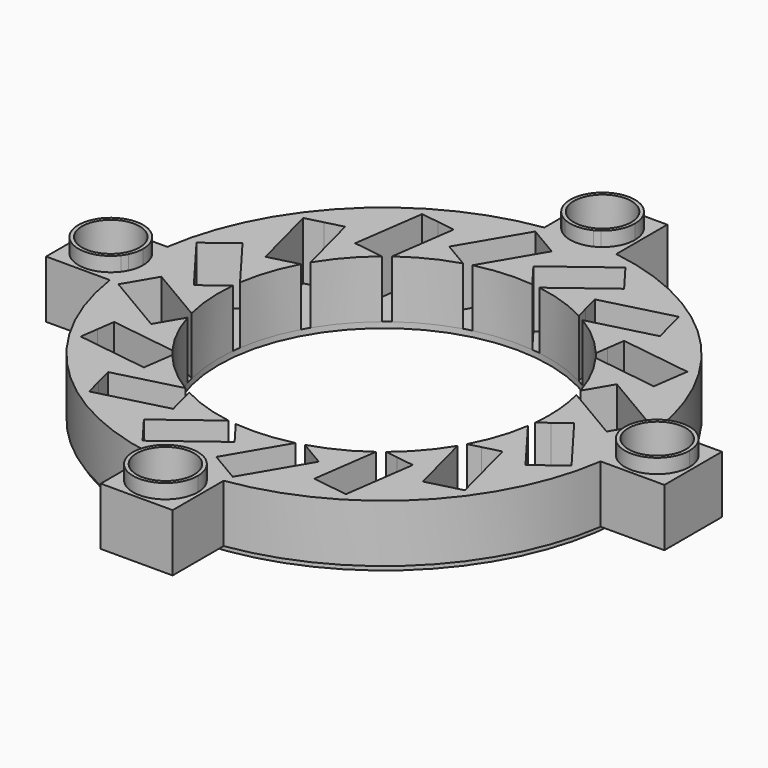
from build123d import *

# Parameters (mm, degrees)
F1_R     = 23
F2_DEPTH = 8
F1_R_2   = 4
F3_DEPTH = 10
F4_DEPTH = 0.8
F5_DEPTH = 25


# Not quite as in the source:
# - a feature names something its author has since deleted; it is built from what else it names


with BuildPart() as f2:
    # F1 (on Top) → F2 (new body)
    with BuildSketch(Plane.XY):
        with BuildLine():
            ThreePointArc((-33.9440789474, -1.9492317499), (-34.1514000153, -2.3320116118), (-34.3947368421, -2.6929681696))
            ThreePointArc((-34.3947368421, -2.6929681696), (-34.2846582705, -3.8486630504), (-34.1357583774, -5))
            ThreePointArc((-34.1357583774, -5), (-24.3951839509, -24.3951839509), (-5, -34.1357583774))
            ThreePointArc((-5, -34.1357583774), (-3.8486630504, -34.2846582705), (-2.6929681696, -34.3947368421))
            ThreePointArc((-2.6929681696, -34.3947368421), (-2.3320116118, -34.1514000153), (-1.9492317499, -33.9440789474))
            ThreePointArc((-1.9492317499, -33.9440789474), (-24.0416305603, -24.0416305603), (-33.9440789474, -1.9492317499))
        make_face()
        with BuildLine():
            ThreePointArc((-34.1357583774, -5), (-34.2846582705, -3.8486630504), (-34.3947368421, -2.6929681696))
            ThreePointArc((-34.3947368421, -2.6929681696), (-42.5, 0), (-34.3947368421, 2.6929681696))
            ThreePointArc((-34.3947368421, 2.6929681696), (-34.2846582705, 3.8486630504), (-34.1357583774, 5))
            Line((-34.1357583774, 5), (-43, 5))
            Line((-43, 5), (-43, 0))
            Line((-43, 0), (-43, -5))
            Line((-43, -5), (-34.1357583774, -5))
        make_face()
        with BuildLine():
            ThreePointArc((-34.1357583774, 5), (-34.2846582705, 3.8486630504), (-34.3947368421, 2.6929681696))
            ThreePointArc((-34.3947368421, 2.6929681696), (-34.1514000153, 2.3320116118), (-33.9440789474, 1.9492317499))
            ThreePointArc((-33.9440789474, 1.9492317499), (-24.0416305603, 24.0416305603), (-1.9492317499, 33.9440789474))
            ThreePointArc((-1.9492317499, 33.9440789474), (-2.3320116118, 34.1514000153), (-2.6929681696, 34.3947368421))
            ThreePointArc((-2.6929681696, 34.3947368421), (-3.8486630504, 34.2846582705), (-5, 34.1357583774))
            ThreePointArc((-5, 34.1357583774), (-24.3951839509, 24.3951839509), (-34.1357583774, 5))
        make_face()
        with BuildLine():
            ThreePointArc((-2.6929681696, -34.3947368421), (-3.8486630504, -34.2846582705), (-5, -34.1357583774))
            Line((-5, -34.1357583774), (-5, -43))
            Line((-5, -43), (0, -43))
            Line((0, -43), (5, -43))
            Line((5, -43), (5, -34.1357583774))
            ThreePointArc((5, -34.1357583774), (3.8486630504, -34.2846582705), (2.6929681696, -34.3947368421))
            ThreePointArc((2.6929681696, -34.3947368421), (4.022956423, -35.9836117392), (4.5, -38))
            ThreePointArc((4.5, -38), (-2.0163882608, -42.022956423), (-2.6929681696, -34.3947368421))
        make_face()
        with BuildLine():
            Line((-5, 43), (-5, 34.1357583774))
            ThreePointArc((-5, 34.1357583774), (-3.8486630504, 34.2846582705), (-2.6929681696, 34.3947368421))
            ThreePointArc((-2.6929681696, 34.3947368421), (-4.2704615799, 39.4188579544), (0, 42.5))
            Line((0, 42.5), (0, 43))
            Line((0, 43), (-5, 43))
        make_face()
        with BuildLine():
            ThreePointArc((33.9440789474, -1.9492317499), (24.0416305603, -24.0416305603), (1.9492317499, -33.9440789474))
            ThreePointArc((1.9492317499, -33.9440789474), (2.3320116118, -34.1514000153), (2.6929681696, -34.3947368421))
            ThreePointArc((2.6929681696, -34.3947368421), (3.8486630504, -34.2846582705), (5, -34.1357583774))
            ThreePointArc((5, -34.1357583774), (24.3951839509, -24.3951839509), (34.1357583774, -5))
            ThreePointArc((34.1357583774, -5), (34.2846582705, -3.8486630504), (34.3947368421, -2.6929681696))
            ThreePointArc((34.3947368421, -2.6929681696), (34.1514000153, -2.3320116118), (33.9440789474, -1.9492317499))
        make_face()
        with BuildLine():
            ThreePointArc((2.6929681696, 34.3947368421), (2.3320116118, 34.1514000153), (1.9492317499, 33.9440789474))
            ThreePointArc((1.9492317499, 33.9440789474), (24.0416305603, 24.0416305603), (33.9440789474, 1.9492317499))
            ThreePointArc((33.9440789474, 1.9492317499), (34.1514000153, 2.3320116118), (34.3947368421, 2.6929681696))
            ThreePointArc((34.3947368421, 2.6929681696), (34.2846582705, 3.8486630504), (34.1357583774, 5))
            ThreePointArc((34.1357583774, 5), (24.3951839509, 24.3951839509), (5, 34.1357583774))
            ThreePointArc((5, 34.1357583774), (3.8486630504, 34.2846582705), (2.6929681696, 34.3947368421))
        make_face()
        with BuildLine():
            Line((0, 43), (0, 42.5))
            ThreePointArc((0, 42.5), (3.1819805153, 41.1819805153), (4.5, 38))
            ThreePointArc((4.5, 38), (4.022956423, 35.9836117392), (2.6929681696, 34.3947368421))
            ThreePointArc((2.6929681696, 34.3947368421), (3.8486630504, 34.2846582705), (5, 34.1357583774))
            Line((5, 34.1357583774), (5, 43))
            Line((5, 43), (0, 43))
        make_face()
        with BuildLine():
            ThreePointArc((42.5, 0), (39.4188579544, -4.2704615799), (34.3947368421, -2.6929681696))
            ThreePointArc((34.3947368421, -2.6929681696), (34.2846582705, -3.8486630504), (34.1357583774, -5))
            Line((34.1357583774, -5), (43, -5))
            Line((43, -5), (43, 0))
            Line((43, 0), (43, 5))
            Line((43, 5), (34.1357583774, 5))
            ThreePointArc((34.1357583774, 5), (34.2846582705, 3.8486630504), (34.3947368421, 2.6929681696))
            ThreePointArc((34.3947368421, 2.6929681696), (39.4188579544, 4.2704615799), (42.5, 0))
        make_face()
        with BuildLine():
            ThreePointArc((-33.5, 0), (-33.6124240897, -0.9995887312), (-33.9440789474, -1.9492317499))
            ThreePointArc((-33.9440789474, -1.9492317499), (-24.0416305603, -24.0416305603), (-1.9492317499, -33.9440789474))
            ThreePointArc((-1.9492317499, -33.9440789474), (0, -33.5), (1.9492317499, -33.9440789474))
            ThreePointArc((1.9492317499, -33.9440789474), (24.0416305603, -24.0416305603), (33.9440789474, -1.9492317499))
            ThreePointArc((33.9440789474, -1.9492317499), (33.5, 0), (33.9440789474, 1.9492317499))
            ThreePointArc((33.9440789474, 1.9492317499), (24.0416305603, 24.0416305603), (1.9492317499, 33.9440789474))
            ThreePointArc((1.9492317499, 33.9440789474), (0, 33.5), (-1.9492317499, 33.9440789474))
            ThreePointArc((-1.9492317499, 33.9440789474), (-24.0416305603, 24.0416305603), (-33.9440789474, 1.9492317499))
            ThreePointArc((-33.9440789474, 1.9492317499), (-33.6124240897, 0.9995887312), (-33.5, 0))
        make_face()
        Circle(F1_R, mode=Mode.SUBTRACT)
    extrude(amount=F2_DEPTH)

    # F1 (on Top) → F3 (join)
    with BuildSketch(Plane.XY):
        with BuildLine():
            ThreePointArc((33.9440789474, 1.9492317499), (33.5, 0), (33.9440789474, -1.9492317499))
            ThreePointArc((33.9440789474, -1.9492317499), (34.1514000153, -2.3320116118), (34.3947368421, -2.6929681696))
            ThreePointArc((34.3947368421, -2.6929681696), (39.4188579544, -4.2704615799), (42.5, 0))
            ThreePointArc((42.5, 0), (39.4188579544, 4.2704615799), (34.3947368421, 2.6929681696))
            ThreePointArc((34.3947368421, 2.6929681696), (34.1514000153, 2.3320116118), (33.9440789474, 1.9492317499))
        make_face()
        with Locations((38, 0)):
            Circle(F1_R_2, mode=Mode.SUBTRACT)
        with BuildLine():
            ThreePointArc((1.9492317499, -33.9440789474), (0, -33.5), (-1.9492317499, -33.9440789474))
            ThreePointArc((-1.9492317499, -33.9440789474), (-2.3320116118, -34.1514000153), (-2.6929681696, -34.3947368421))
            ThreePointArc((-2.6929681696, -34.3947368421), (-2.0163882608, -42.022956423), (4.5, -38))
            ThreePointArc((4.5, -38), (4.022956423, -35.9836117392), (2.6929681696, -34.3947368421))
            ThreePointArc((2.6929681696, -34.3947368421), (2.3320116118, -34.1514000153), (1.9492317499, -33.9440789474))
        make_face()
        with Locations((0, -38)):
            Circle(F1_R_2, mode=Mode.SUBTRACT)
        with BuildLine():
            ThreePointArc((-34.3947368421, 2.6929681696), (-42.5, 0), (-34.3947368421, -2.6929681696))
            ThreePointArc((-34.3947368421, -2.6929681696), (-34.1514000153, -2.3320116118), (-33.9440789474, -1.9492317499))
            ThreePointArc((-33.9440789474, -1.9492317499), (-33.6124240897, -0.9995887312), (-33.5, 0))
            ThreePointArc((-33.5, 0), (-33.6124240897, 0.9995887312), (-33.9440789474, 1.9492317499))
            ThreePointArc((-33.9440789474, 1.9492317499), (-34.1514000153, 2.3320116118), (-34.3947368421, 2.6929681696))
        make_face()
        with Locations((-38, 0)):
            Circle(F1_R_2, mode=Mode.SUBTRACT)
        with BuildLine():
            ThreePointArc((-2.6929681696, 34.3947368421), (-2.3320116118, 34.1514000153), (-1.9492317499, 33.9440789474))
            ThreePointArc((-1.9492317499, 33.9440789474), (0, 33.5), (1.9492317499, 33.9440789474))
            ThreePointArc((1.9492317499, 33.9440789474), (2.3320116118, 34.1514000153), (2.6929681696, 34.3947368421))
            ThreePointArc((2.6929681696, 34.3947368421), (4.022956423, 35.9836117392), (4.5, 38))
            ThreePointArc((4.5, 38), (3.1819805153, 41.1819805153), (0, 42.5))
            ThreePointArc((0, 42.5), (-4.2704615799, 39.4188579544), (-2.6929681696, 34.3947368421))
        make_face()
        with Locations((0, 38)):
            Circle(F1_R_2, mode=Mode.SUBTRACT)
    extrude(amount=F3_DEPTH)

    # F1 (on Top) → F4 (join)
    with BuildSketch(Plane.XY):
        with BuildLine():
            ThreePointArc((-33.5, 0), (-33.6124240897, -0.9995887312), (-33.9440789474, -1.9492317499))
            ThreePointArc((-33.9440789474, -1.9492317499), (-24.0416305603, -24.0416305603), (-1.9492317499, -33.9440789474))
            ThreePointArc((-1.9492317499, -33.9440789474), (0, -33.5), (1.9492317499, -33.9440789474))
            ThreePointArc((1.9492317499, -33.9440789474), (24.0416305603, -24.0416305603), (33.9440789474, -1.9492317499))
            ThreePointArc((33.9440789474, -1.9492317499), (33.5, 0), (33.9440789474, 1.9492317499))
            ThreePointArc((33.9440789474, 1.9492317499), (24.0416305603, 24.0416305603), (1.9492317499, 33.9440789474))
            ThreePointArc((1.9492317499, 33.9440789474), (0, 33.5), (-1.9492317499, 33.9440789474))
            ThreePointArc((-1.9492317499, 33.9440789474), (-24.0416305603, 24.0416305603), (-33.9440789474, 1.9492317499))
            ThreePointArc((-33.9440789474, 1.9492317499), (-33.6124240897, 0.9995887312), (-33.5, 0))
        make_face()
        Circle(F1_R, mode=Mode.SUBTRACT)
    extrude(amount=-F4_DEPTH)

    # F0 (on Top) → F5 (cut)
    with BuildSketch(Plane.XY):
        with BuildLine():
            ThreePointArc((-14.5432880163, 17.8183269045), (-14.1135037547, 18.1606445857), (-13.6756650336, 18.4925981379))
            Line((-13.6756650336, 18.4925981379), (-12.3936663154, 27.6144930015))
            Line((-12.3936663154, 27.6144930015), (-14.8693364872, 27.9624257539))
            Line((-14.8693364872, 27.9624257539), (-17.3450066591, 28.3103585063))
            Line((-17.3450066591, 28.3103585063), (-18.7367376687, 18.4076778189))
            Line((-18.7367376687, 18.4076778189), (-16.2610674968, 18.0597450665))
            Line((-16.2610674968, 18.0597450665), (-14.5432880163, 17.8183269045))
        make_face()
        with BuildLine():
            ThreePointArc((-6.6174676349, 22.0274629066), (-6.0893994469, 22.1792518895), (-5.5578560893, 22.3183833575))
            Line((-5.5578560893, 22.3183833575), (-0.8826456767, 30.2553156499))
            Line((-0.8826456767, 30.2553156499), (-3.0367185778, 31.5241615573))
            Line((-3.0367185778, 31.5241615573), (-5.1907914789, 32.7930074647))
            Line((-5.1907914789, 32.7930074647), (-10.2661751085, 24.1767158603))
            Line((-10.2661751085, 24.1767158603), (-8.1121022074, 22.9078699529))
            Line((-8.1121022074, 22.9078699529), (-6.6174676349, 22.0274629066))
        make_face()
        with BuildLine():
            ThreePointArc((2.3158022064, 22.8831173606), (2.861760726, 22.8212691485), (3.4060860626, 22.7463970275))
            Line((3.4060860626, 22.7463970275), (10.762749765, 28.2900407558))
            Line((10.762749765, 28.2900407558), (9.2582122071, 30.2866295309))
            Line((9.2582122071, 30.2866295309), (7.7536746492, 32.283218306))
            Line((7.7536746492, 32.283218306), (-0.2326804512, 26.2650680745))
            Line((-0.2326804512, 26.2650680745), (1.2718571067, 24.2684792994))
            Line((1.2718571067, 24.2684792994), (2.3158022064, 22.8831173606))
        make_face()
        with BuildLine():
            ThreePointArc((10.8965121547, 20.2550246325), (11.3772437704, 19.988955055), (11.8514824876, 19.7114779468))
            Line((11.8514824876, 19.7114779468), (20.7696141196, 22.0178636064))
            Line((20.7696141196, 22.0178636064), (20.1436641095, 24.4382327073))
            Line((20.1436641095, 24.4382327073), (19.5177140993, 26.8586018083))
            Line((19.5177140993, 26.8586018083), (9.8362376955, 24.3548017677))
            Line((9.8362376955, 24.3548017677), (10.4621877057, 21.9344326668))
            Line((10.4621877057, 21.9344326668), (10.8965121547, 20.2550246325))
        make_face()
        with BuildLine():
            ThreePointArc((17.8183269045, 14.5432880163), (18.1606445857, 14.1135037547), (18.4925981379, 13.6756650336))
            Line((18.4925981379, 13.6756650336), (27.6144930015, 12.3936663154))
            Line((27.6144930015, 12.3936663154), (27.9624257539, 14.8693364872))
            Line((27.9624257539, 14.8693364872), (28.3103585063, 17.3450066591))
            Line((28.3103585063, 17.3450066591), (18.4076778189, 18.7367376687))
            Line((18.4076778189, 18.7367376687), (18.0597450665, 16.2610674968))
            Line((18.0597450665, 16.2610674968), (17.8183269045, 14.5432880163))
        make_face()
        with BuildLine():
            ThreePointArc((22.0274629066, 6.6174676349), (22.1792518895, 6.0893994469), (22.3183833575, 5.5578560893))
            Line((22.3183833575, 5.5578560893), (30.2553156499, 0.8826456767))
            Line((30.2553156499, 0.8826456767), (31.5241615573, 3.0367185778))
            Line((31.5241615573, 3.0367185778), (32.7930074647, 5.1907914789))
            Line((32.7930074647, 5.1907914789), (24.1767158603, 10.2661751085))
            Line((24.1767158603, 10.2661751085), (22.9078699529, 8.1121022074))
            Line((22.9078699529, 8.1121022074), (22.0274629066, 6.6174676349))
        make_face()
        with BuildLine():
            Line((24.2684792994, -1.2718571067), (22.8831173606, -2.3158022064))
            ThreePointArc((22.8831173606, -2.3158022064), (22.8212691485, -2.861760726), (22.7463970275, -3.4060860626))
            Line((22.7463970275, -3.4060860626), (28.2900407558, -10.762749765))
            Line((28.2900407558, -10.762749765), (30.2866295309, -9.2582122071))
            Line((30.2866295309, -9.2582122071), (32.283218306, -7.7536746492))
            Line((32.283218306, -7.7536746492), (26.2650680745, 0.2326804512))
            Line((26.2650680745, 0.2326804512), (24.2684792994, -1.2718571067))
        make_face()
        with BuildLine():
            Line((21.9344326668, -10.4621877057), (20.2550246325, -10.8965121547))
            ThreePointArc((20.2550246325, -10.8965121547), (19.988955055, -11.3772437704), (19.7114779468, -11.8514824876))
            Line((19.7114779468, -11.8514824876), (22.0178636064, -20.7696141196))
            Line((22.0178636064, -20.7696141196), (24.4382327073, -20.1436641095))
            Line((24.4382327073, -20.1436641095), (26.8586018083, -19.5177140993))
            Line((26.8586018083, -19.5177140993), (24.3548017677, -9.8362376955))
            Line((24.3548017677, -9.8362376955), (21.9344326668, -10.4621877057))
        make_face()
        with BuildLine():
            Line((16.2610674968, -18.0597450665), (14.5432880163, -17.8183269045))
            ThreePointArc((14.5432880163, -17.8183269045), (14.1135037547, -18.1606445857), (13.6756650336, -18.4925981379))
            Line((13.6756650336, -18.4925981379), (12.3936663154, -27.6144930015))
            Line((12.3936663154, -27.6144930015), (14.8693364872, -27.9624257539))
            Line((14.8693364872, -27.9624257539), (17.3450066591, -28.3103585063))
            Line((17.3450066591, -28.3103585063), (18.7367376687, -18.4076778189))
            Line((18.7367376687, -18.4076778189), (16.2610674968, -18.0597450665))
        make_face()
        with BuildLine():
            Line((8.1121022074, -22.9078699529), (6.6174676349, -22.0274629066))
            ThreePointArc((6.6174676349, -22.0274629066), (6.0893994469, -22.1792518895), (5.5578560893, -22.3183833575))
            Line((5.5578560893, -22.3183833575), (0.8826456767, -30.2553156499))
            Line((0.8826456767, -30.2553156499), (3.0367185778, -31.5241615573))
            Line((3.0367185778, -31.5241615573), (5.1907914789, -32.7930074647))
            Line((5.1907914789, -32.7930074647), (10.2661751085, -24.1767158603))
            Line((10.2661751085, -24.1767158603), (8.1121022074, -22.9078699529))
        make_face()
        with BuildLine():
            Line((-1.2718571067, -24.2684792994), (-2.3158022064, -22.8831173606))
            ThreePointArc((-2.3158022064, -22.8831173606), (-2.861760726, -22.8212691485), (-3.4060860626, -22.7463970275))
            Line((-3.4060860626, -22.7463970275), (-10.762749765, -28.2900407558))
            Line((-10.762749765, -28.2900407558), (-9.2582122071, -30.2866295309))
            Line((-9.2582122071, -30.2866295309), (-7.7536746492, -32.283218306))
            Line((-7.7536746492, -32.283218306), (0.2326804512, -26.2650680745))
            Line((0.2326804512, -26.2650680745), (-1.2718571067, -24.2684792994))
        make_face()
        with BuildLine():
            Line((-10.4621877057, -21.9344326668), (-10.8965121547, -20.2550246325))
            ThreePointArc((-10.8965121547, -20.2550246325), (-11.3772437704, -19.988955055), (-11.8514824876, -19.7114779468))
            Line((-11.8514824876, -19.7114779468), (-20.7696141196, -22.0178636064))
            Line((-20.7696141196, -22.0178636064), (-20.1436641095, -24.4382327073))
            Line((-20.1436641095, -24.4382327073), (-19.5177140993, -26.8586018083))
            Line((-19.5177140993, -26.8586018083), (-9.8362376955, -24.3548017677))
            Line((-9.8362376955, -24.3548017677), (-10.4621877057, -21.9344326668))
        make_face()
        with BuildLine():
            Line((-18.0597450665, -16.2610674968), (-17.8183269045, -14.5432880163))
            ThreePointArc((-17.8183269045, -14.5432880163), (-18.1606445857, -14.1135037547), (-18.4925981379, -13.6756650336))
            Line((-18.4925981379, -13.6756650336), (-27.6144930015, -12.3936663154))
            Line((-27.6144930015, -12.3936663154), (-27.9624257539, -14.8693364872))
            Line((-27.9624257539, -14.8693364872), (-28.3103585063, -17.3450066591))
            Line((-28.3103585063, -17.3450066591), (-18.4076778189, -18.7367376687))
            Line((-18.4076778189, -18.7367376687), (-18.0597450665, -16.2610674968))
        make_face()
        with BuildLine():
            Line((-22.9078699529, -8.1121022074), (-22.0274629066, -6.6174676349))
            ThreePointArc((-22.0274629066, -6.6174676349), (-22.1792518895, -6.0893994469), (-22.3183833575, -5.5578560893))
            Line((-22.3183833575, -5.5578560893), (-30.2553156499, -0.8826456767))
            Line((-30.2553156499, -0.8826456767), (-31.5241615573, -3.0367185778))
            Line((-31.5241615573, -3.0367185778), (-32.7930074647, -5.1907914789))
            Line((-32.7930074647, -5.1907914789), (-24.1767158603, -10.2661751085))
            Line((-24.1767158603, -10.2661751085), (-22.9078699529, -8.1121022074))
        make_face()
        with BuildLine():
            ThreePointArc((-22.8831173606, 2.3158022064), (-22.8212691485, 2.861760726), (-22.7463970275, 3.4060860626))
            Line((-22.7463970275, 3.4060860626), (-28.2900407558, 10.762749765))
            Line((-28.2900407558, 10.762749765), (-30.2866295309, 9.2582122071))
            Line((-30.2866295309, 9.2582122071), (-32.283218306, 7.7536746492))
            Line((-32.283218306, 7.7536746492), (-26.2650680745, -0.2326804512))
            Line((-26.2650680745, -0.2326804512), (-24.2684792994, 1.2718571067))
            Line((-24.2684792994, 1.2718571067), (-22.8831173606, 2.3158022064))
        make_face()
        with BuildLine():
            ThreePointArc((-20.2550246325, 10.8965121547), (-19.988955055, 11.3772437704), (-19.7114779468, 11.8514824876))
            Line((-19.7114779468, 11.8514824876), (-22.0178636064, 20.7696141196))
            Line((-22.0178636064, 20.7696141196), (-24.4382327073, 20.1436641095))
            Line((-24.4382327073, 20.1436641095), (-26.8586018083, 19.5177140993))
            Line((-26.8586018083, 19.5177140993), (-24.3548017677, 9.8362376955))
            Line((-24.3548017677, 9.8362376955), (-21.9344326668, 10.4621877057))
            Line((-21.9344326668, 10.4621877057), (-20.2550246325, 10.8965121547))
        make_face()
    extrude(amount=F5_DEPTH, mode=Mode.SUBTRACT)


solid = f2.part
